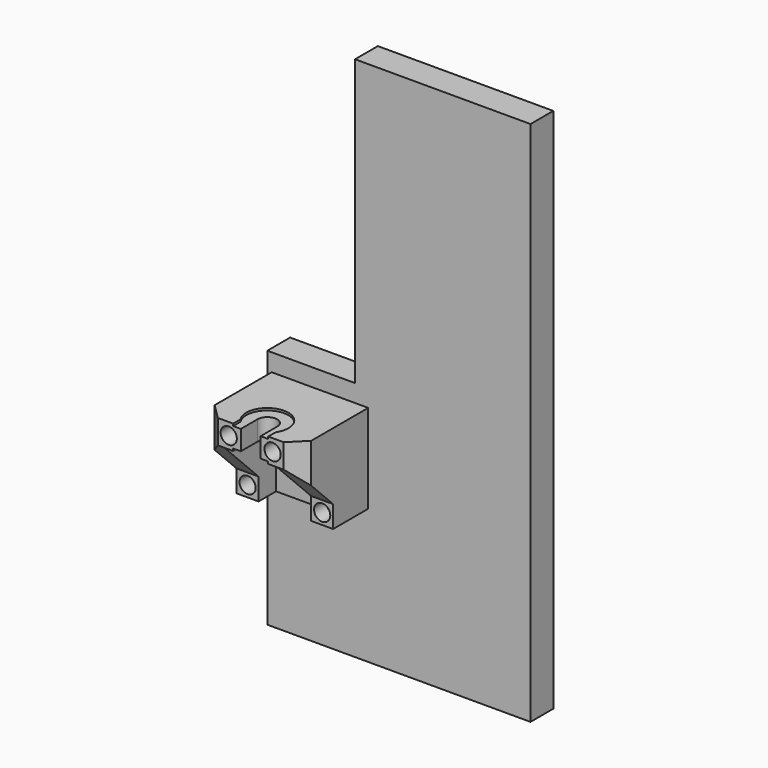
from build123d import *

# Parameters (mm, degrees)
F1_DEPTH  = 13
F2_D      = 3.5
F3_R      = 3.7
F3_W      = 24
F3_H      = 29.5
F3_R_2    = 2.1
F3_R_3    = 1.75
F4_DEPTH  = 39.5
F5_DEPTH  = 39.501
F6_START  = 30
F6_DEPTH  = 9.501
F7_START  = 13
F7_DEPTH  = 26.501
F9_DEPTH  = 10
F11_DEPTH = 118.001
F12_DEPTH = 102.001
F13_DEPTH = 1
F14_START = -10
F14_DEPTH = 92.001
F15_SIZE  = 7


with BuildPart() as f1:
    # F0 (on Front) → F1 (new body)
    with BuildSketch(Plane.XZ):
        Polygon((-18.6688979508, 54.3871098008), (-58.6688979508, 54.3871098008), (-58.6688979508, -55.6128901992), (61.3311020492, -55.6128901992), (61.3311020492, 184.3871098008), (-18.6688979508, 184.3871098008), align=None)
    extrude(amount=F1_DEPTH)

    # F2 (through all)
    with Locations(Plane(origin=(0, 0, 0), x_dir=(1, 0, 0), z_dir=(0, 1, 0))):
        with Locations((-44.6688979508, -40.8871098008), (-24.6688979508, -40.8871098008), (-51.6688979508, -10.8871098008), (-17.6688979508, -10.8871098008)):
            Hole(F2_D / 2)


with BuildPart() as f4:
    # F3 (on face) → F4 (new body)
    with BuildSketch(Plane.XZ.offset(13)):
        Polygon((-22.6688979508, 5.8871098008), (-12.6688979508, 5.8871098008), (-12.6688979508, 46.3871098008), (-56.6688979508, 46.3871098008), (-56.6688979508, 5.8871098008), (-46.6688979508, 5.8871098008), (-46.6688979508, 35.3871098008), (-22.6688979508, 35.3871098008), align=None)
        with Locations((-51.6688979508, 10.8871098008)):
            Circle(F3_R, mode=Mode.SUBTRACT)
        with Locations((-44.6688979508, 40.8871098008)):
            Circle(F3_R, mode=Mode.SUBTRACT)
        with Locations((-17.6688979508, 10.8871098008)):
            Circle(F3_R, mode=Mode.SUBTRACT)
        with Locations((-24.6688979508, 40.8871098008)):
            Circle(F3_R, mode=Mode.SUBTRACT)
        with Locations((-34.6688979508, 20.6371098008)):
            Rectangle(F3_W, F3_H)
        with Locations((-44.6688979508, 40.8871098008)):
            Circle(F3_R)
        with Locations((-44.6688979508, 40.8871098008)):
            Circle(F3_R_2, mode=Mode.SUBTRACT)
        with Locations((-24.6688979508, 40.8871098008)):
            Circle(F3_R)
        with Locations((-24.6688979508, 40.8871098008)):
            Circle(F3_R_2, mode=Mode.SUBTRACT)
        with Locations((-51.6688979508, 10.8871098008)):
            Circle(F3_R)
        with Locations((-51.6688979508, 10.8871098008)):
            Circle(F3_R_2, mode=Mode.SUBTRACT)
        with Locations((-17.6688979508, 10.8871098008)):
            Circle(F3_R)
        with Locations((-17.6688979508, 10.8871098008)):
            Circle(F3_R_2, mode=Mode.SUBTRACT)
        with Locations((-17.6688979508, 10.8871098008)):
            Circle(F3_R_2)
        with Locations((-17.6688979508, 10.8871098008)):
            Circle(F3_R_3, mode=Mode.SUBTRACT)
        with Locations((-51.6688979508, 10.8871098008)):
            Circle(F3_R_2)
        with Locations((-51.6688979508, 10.8871098008)):
            Circle(F3_R_3, mode=Mode.SUBTRACT)
        with Locations((-44.6688979508, 40.8871098008)):
            Circle(F3_R_2)
        with Locations((-44.6688979508, 40.8871098008)):
            Circle(F3_R_3, mode=Mode.SUBTRACT)
        with Locations((-24.6688979508, 40.8871098008)):
            Circle(F3_R_2)
        with Locations((-24.6688979508, 40.8871098008)):
            Circle(F3_R_3, mode=Mode.SUBTRACT)
    extrude(amount=F4_DEPTH)

    # F3 (on face) → F5 (cut, through all)
    with BuildSketch(Plane.XZ.offset(13)):
        with Locations((-34.6688979508, 20.6371098008)):
            Rectangle(F3_W, F3_H)
        with Locations((-17.6688979508, 10.8871098008)):
            Circle(F3_R_2)
        with Locations((-17.6688979508, 10.8871098008)):
            Circle(F3_R_3, mode=Mode.SUBTRACT)
        with Locations((-51.6688979508, 10.8871098008)):
            Circle(F3_R_2)
        with Locations((-51.6688979508, 10.8871098008)):
            Circle(F3_R_3, mode=Mode.SUBTRACT)
        with Locations((-44.6688979508, 40.8871098008)):
            Circle(F3_R_2)
        with Locations((-44.6688979508, 40.8871098008)):
            Circle(F3_R_3, mode=Mode.SUBTRACT)
        with Locations((-24.6688979508, 40.8871098008)):
            Circle(F3_R_2)
        with Locations((-24.6688979508, 40.8871098008)):
            Circle(F3_R_3, mode=Mode.SUBTRACT)
    extrude(amount=F5_DEPTH, mode=Mode.SUBTRACT)

    # F3 (on face) → F6 (cut)
    with BuildSketch(Plane.XZ.offset(13).offset(F6_START)):
        with Locations((-44.6688979508, 40.8871098008)):
            Circle(F3_R)
        with Locations((-44.6688979508, 40.8871098008)):
            Circle(F3_R_2, mode=Mode.SUBTRACT)
        with Locations((-24.6688979508, 40.8871098008)):
            Circle(F3_R)
        with Locations((-24.6688979508, 40.8871098008)):
            Circle(F3_R_2, mode=Mode.SUBTRACT)
    extrude(amount=F6_DEPTH, mode=Mode.SUBTRACT)

    # F3 (on face) → F7 (cut)
    with BuildSketch(Plane.XZ.offset(13).offset(F7_START)):
        with Locations((-17.6688979508, 10.8871098008)):
            Circle(F3_R)
        with Locations((-17.6688979508, 10.8871098008)):
            Circle(F3_R_2, mode=Mode.SUBTRACT)
        with Locations((-51.6688979508, 10.8871098008)):
            Circle(F3_R)
        with Locations((-51.6688979508, 10.8871098008)):
            Circle(F3_R_2, mode=Mode.SUBTRACT)
    extrude(amount=F7_DEPTH, mode=Mode.SUBTRACT)

    # F3 (on face) → F9 (join)
    with BuildSketch(Plane.XZ.offset(13)):
        with Locations((-34.6688979508, 20.6371098008)):
            Rectangle(F3_W, F3_H)
        with Locations((-51.6688979508, 10.8871098008)):
            Circle(F3_R)
        with Locations((-51.6688979508, 10.8871098008)):
            Circle(F3_R_2, mode=Mode.SUBTRACT)
        with Locations((-17.6688979508, 10.8871098008)):
            Circle(F3_R)
        with Locations((-17.6688979508, 10.8871098008)):
            Circle(F3_R_2, mode=Mode.SUBTRACT)
    extrude(amount=F9_DEPTH)

    # F10 (on face) → F11 (cut, through all)
    with BuildSketch(Plane(origin=(-56.6688979508, 0, 0), x_dir=(0, -1, 0), z_dir=(-1, 0, 0))):
        Polygon((52.5, 5.8871098008), (52.5, 35.3871098008), (33, 15.8871098008), (33, 5.8871098008), align=None)
    extrude(amount=-F11_DEPTH, mode=Mode.SUBTRACT)

    # F8 (on face) → F12 (cut, through all)
    with BuildSketch(Plane.XY.offset(46.3871098008)):
        with BuildLine():
            Line((-39.1688979508, -52.5), (-30.1688979508, -52.5))
            Line((-30.1688979508, -52.5), (-30.1688979508, -43))
            ThreePointArc((-30.1688979508, -43), (-34.6688979508, -38.5), (-39.1688979508, -43))
            Line((-39.1688979508, -43), (-39.1688979508, -52.5))
        make_face()
    extrude(amount=-F12_DEPTH, mode=Mode.SUBTRACT)

    # F8 (on face) → F13 (cut)
    with BuildSketch(Plane.XY.offset(46.3871098008)):
        with BuildLine():
            Line((-26.6688979508, -52.5), (-26.6688979508, -48.3065996646))
            ThreePointArc((-26.6688979508, -48.3065996646), (-34.6688979508, -33.4), (-42.6688979508, -48.3065996646))
            Line((-42.6688979508, -48.3065996646), (-42.6688979508, -52.5))
            Line((-42.6688979508, -52.5), (-39.1688979508, -52.5))
            Line((-39.1688979508, -52.5), (-39.1688979508, -43))
            ThreePointArc((-39.1688979508, -43), (-34.6688979508, -38.5), (-30.1688979508, -43))
            Line((-30.1688979508, -43), (-30.1688979508, -52.5))
            Line((-30.1688979508, -52.5), (-26.6688979508, -52.5))
        make_face()
    extrude(amount=-F13_DEPTH, mode=Mode.SUBTRACT)

    # F8 (on face) → F14 (cut)
    with BuildSketch(Plane.XY.offset(46.3871098008).offset(F14_START)):
        with BuildLine():
            Line((-26.6688979508, -52.5), (-26.6688979508, -48.3065996646))
            ThreePointArc((-26.6688979508, -48.3065996646), (-34.6688979508, -33.4), (-42.6688979508, -48.3065996646))
            Line((-42.6688979508, -48.3065996646), (-42.6688979508, -52.5))
            Line((-42.6688979508, -52.5), (-39.1688979508, -52.5))
            Line((-39.1688979508, -52.5), (-39.1688979508, -43))
            ThreePointArc((-39.1688979508, -43), (-34.6688979508, -38.5), (-30.1688979508, -43))
            Line((-30.1688979508, -43), (-30.1688979508, -52.5))
            Line((-30.1688979508, -52.5), (-26.6688979508, -52.5))
        make_face()
    extrude(amount=-F14_DEPTH, mode=Mode.SUBTRACT)

    # F15
    f15_edges = [f4.edges().sort_by_distance(p)[0] for p in [
        (-56.668898, -52.5, 40.88711),
        (-12.668898, -52.5, 40.88711),
    ]]
    chamfer(f15_edges, length=F15_SIZE)


solid = Compound([f1.part, f4.part])
